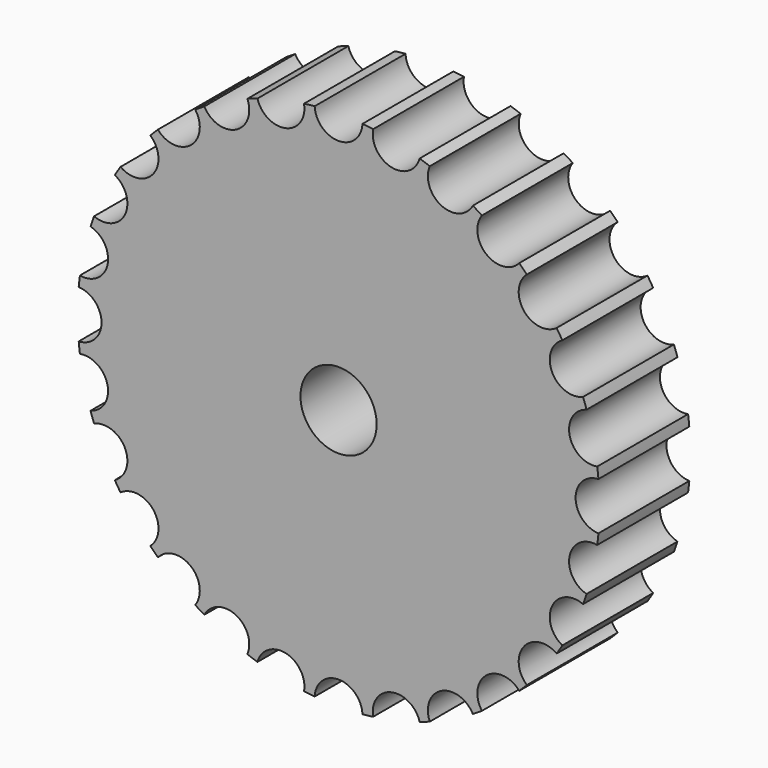
from build123d import *

# Parameters (mm, degrees)
F0_R            = 58.3586225364
F1_DEPTH        = 25.4
F3_DEPTH        = 25.401
F3_COPIES_COUNT = 28
F5_R            = 8.5203865575
F6_DEPTH        = 25.401
F7_T            = -2.54


# Not quite as in the source:
# - a feature of the source that left no trace in its solid (it failed there, or was rolled back) is left out
# - a pattern or mirror of a feature is missing from the dataset's text; its kind, count and spacing are read off the source's solid


with BuildPart() as f1:
    # F0 (on Front) → F1 (new body)
    with BuildSketch(Plane.XZ):
        Circle(F0_R)
    extrude(amount=F1_DEPTH)

    # F2 (on face) → F3 (cut, through all)
    with BuildSketch(Plane.XZ.offset(25.4)):
        with BuildLine():
            ThreePointArc((5.3432300873, 58.1134985746), (0, 58.3586225364), (-5.3432300873, 58.1134985746))
            ThreePointArc((-5.3432300873, 58.1134985746), (0, 53.0097727981), (5.3432300873, 58.1134985746))
        make_face()
    f3 = extrude(amount=-F3_DEPTH, mode=Mode.SUBTRACT)

    # F3_copies: F3 ×28 about axis
    f3_copies_axis = Axis((0, 0, 0), (0, 1, 0))
    for i in range(1, F3_COPIES_COUNT):
        add(f3.rotate(f3_copies_axis, i * 360 / F3_COPIES_COUNT), mode=Mode.SUBTRACT)

    # F5 (on face) → F6 (cut, through all)
    with BuildSketch(Plane.XZ.offset(25.4)):
        Circle(F5_R)
    extrude(amount=-F6_DEPTH, mode=Mode.SUBTRACT)

    # F7
    f7_openings = [f1.faces().sort_by_distance(p)[0] for p in [
        (0, 0, 51.366075),
    ]]
    offset(amount=F7_T, openings=f7_openings)


solid = f1.part
